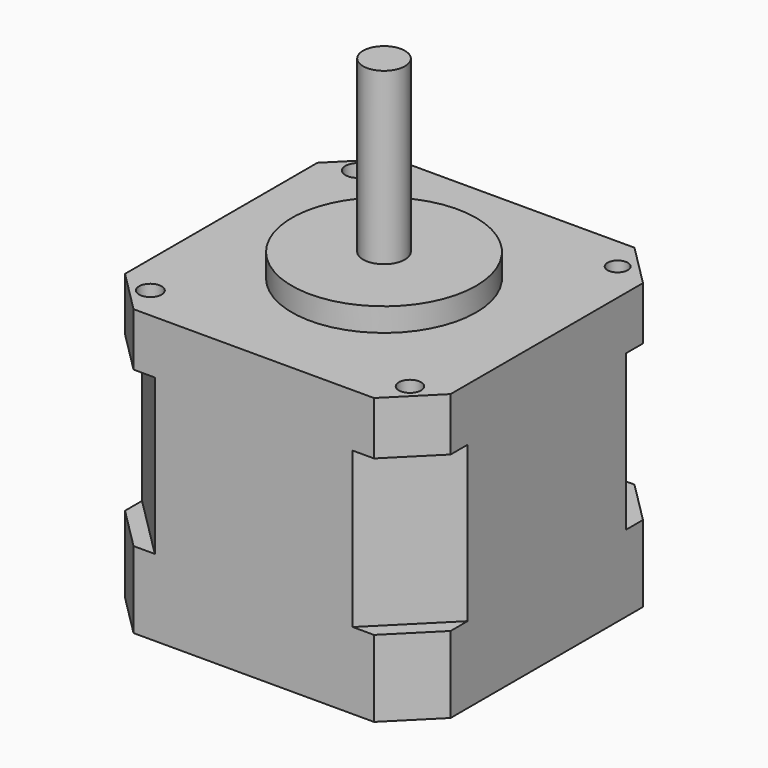
from build123d import *

# Parameters (mm, degrees)
F0_W      = 38.862
F0_H      = 38.862
F1_DEPTH  = 10.668
F2_SIZE   = 7.62
F4_DEPTH  = 6.35
F5_SIZE   = 5.08
F7_DEPTH  = 6.35
F8_R      = 10.9982
F9_DEPTH  = 2.794
F10_R     = 2.5
F11_DEPTH = 20.32
F12_W     = 13.1343230445
F12_H     = 2.3335092461
F13_DEPTH = 10.16
F14_R     = 1.5
F14_R_2   = 1.2067449727
F14_R_3   = 1.3291263225
F14_R_4   = 1.3491824754
F15_DEPTH = 6.35


# Not quite as in the source:
# - a feature names something its author has since deleted; it is built from what else it names


with BuildPart() as f1:
    # F0 (on Top) → F1 (new body, symmetric)
    with BuildSketch(Plane.XY):
        Rectangle(F0_W, F0_H)
    extrude(amount=F1_DEPTH, both=True)

    # F2
    f2_edges = [f1.edges().sort_by_distance(p)[0] for p in [
        (19.431, 19.431, 0),
        (-19.431, 19.431, 0),
        (-19.431, -19.431, 0),
        (19.431, -19.431, 0),
    ]]
    chamfer(f2_edges, length=F2_SIZE)

    # F3 (on face) → F4 (join)
    with BuildSketch(Plane.XY.offset(10.668)):
        Polygon((11.811, 19.431), (-11.811, 19.431), (-19.431, 11.811), (-19.431, -11.811), (-11.811, -19.431), (11.811, -19.431), (19.431, -11.811), (19.431, 11.811), align=None)
        Polygon((19.431, 19.431), (11.811, 19.431), (19.431, 11.811), align=None)
        Polygon((-11.811, 19.431), (-19.431, 19.431), (-19.431, 11.811), align=None)
        Polygon((-11.811, -19.431), (-19.431, -11.811), (-19.431, -19.431), align=None)
        Polygon((19.431, -19.431), (19.431, -11.811), (11.811, -19.431), align=None)
    extrude(amount=F4_DEPTH)

    # F5
    f5_edges = [f1.edges().sort_by_distance(p)[0] for p in [
        (19.431, 19.431, 13.843),
        (-19.431, 19.431, 13.843),
        (-19.431, -19.431, 13.843),
        (19.431, -19.431, 13.843),
    ]]
    chamfer(f5_edges, length=F5_SIZE)

    # F6 (on face) → F7 (join)
    with BuildSketch(Plane(origin=(0, 0, -10.668), x_dir=(1, 0, 0), z_dir=(0, 0, -1))):
        Polygon((-11.811, 19.431), (-14.351, 19.431), (-19.431, 14.351), (-19.431, 11.811), align=None)
        Polygon((14.351, 19.431), (11.811, 19.431), (19.431, 11.811), (19.431, 14.351), align=None)
        Polygon((19.431, -14.351), (19.431, -11.811), (11.811, -19.431), (14.351, -19.431), align=None)
        Polygon((-11.811, -19.431), (-19.431, -11.811), (-19.431, -14.351), (-14.351, -19.431), align=None)
        Polygon((11.811, 19.431), (-11.811, 19.431), (-19.431, 11.811), (-19.431, -11.811), (-11.811, -19.431), (11.811, -19.431), (19.431, -11.811), (19.431, 11.811), align=None)
    extrude(amount=F7_DEPTH)

    # F8 (on face) + F6 (on face) → F9 (join)
    with BuildSketch(Plane.XY.offset(17.018)):
        Circle(F8_R)
    with BuildSketch(Plane(origin=(0, 0, -10.668), x_dir=(1, 0, 0), z_dir=(0, 0, -1))):
        Polygon((14.351, 19.431), (-14.351, 19.431), (-19.431, 14.351), (-19.431, -14.351), (-14.351, -19.431), (14.351, -19.431), (19.431, -14.351), (19.431, 14.351), align=None)
    extrude(amount=F9_DEPTH, dir=(0, 0, 1))

    # F10 (on face) → F11 (join)
    with BuildSketch(Plane.XY.offset(19.812)):
        Circle(F10_R)
    extrude(amount=F11_DEPTH)

    # F12 (on face) → F13 (cut)
    with BuildSketch(Plane.XY.offset(40.132)):
        with Locations((-0.0065014465, 6.166754623)):
            Rectangle(F12_W, F12_H)
    extrude(amount=-F13_DEPTH, mode=Mode.SUBTRACT)

    # F14 (on face) → F15 (cut)
    with BuildSketch(Plane.XY.offset(17.018)):
        with Locations((-15.5, 15.494)):
            Circle(F14_R)
        with Locations((15.494, 15.494)):
            Circle(F14_R_2)
        with Locations((15.494, -15.494)):
            Circle(F14_R_3)
        with Locations((-15.494, -15.494)):
            Circle(F14_R_4)
    extrude(amount=-F15_DEPTH, mode=Mode.SUBTRACT)


solid = f1.part
